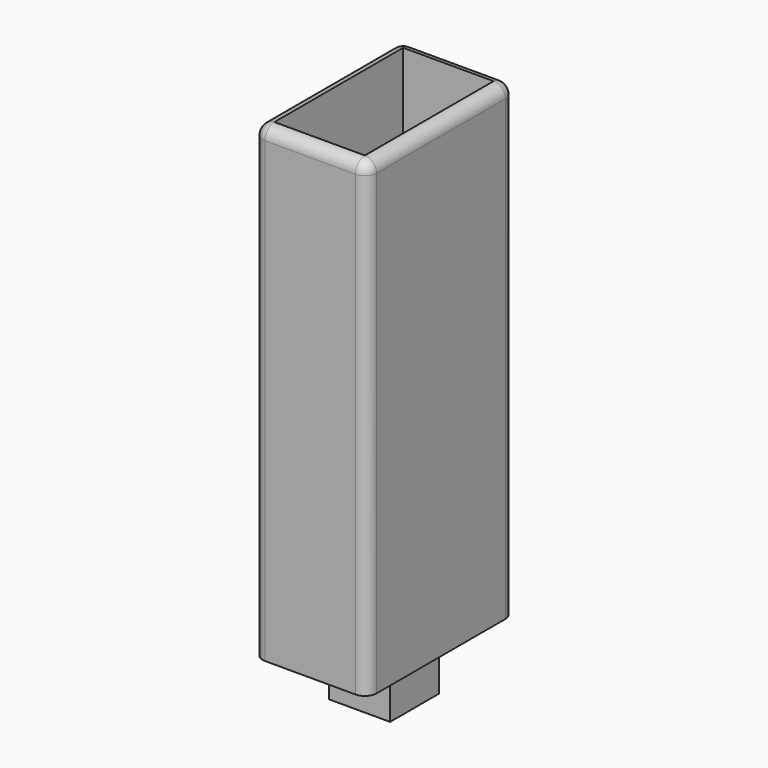
from build123d import *

# Parameters (mm, degrees)
F0_W     = 12.319
F0_H     = 19.939
F1_DEPTH = 50.8
F2_T     = -1.27
F3_R     = 1.26999
F4_W     = 6.604
F4_H     = 6.604
F5_DEPTH = 5.842


# Not quite as in the source:
# - a fillet or chamfer is up to 0.001 mm smaller than in the source, because OpenCascade refuses the exact size


with BuildPart() as f1:
    # F0 (on Top) → F1 (new body)
    with BuildSketch(Plane.XY):
        Rectangle(F0_W, F0_H)
    extrude(amount=F1_DEPTH)

    # F2
    f2_openings = [f1.faces().sort_by_distance(p)[0] for p in [
        (0, 0, 50.8),
    ]]
    offset(amount=F2_T, openings=f2_openings)

    # F3 (radius 1.27 in the source; OpenCascade refuses exactly that, so slightly less here)
    f3_edges = [f1.edges().sort_by_distance(p)[0] for p in [
        (0, -9.9695, 50.8),
        (6.1595, 0, 50.8),
        (0, 9.9695, 50.8),
        (-6.1595, 0, 50.8),
        (-6.1595, -9.9695, 25.4),
        (6.1595, -9.9695, 25.4),
        (6.1595, 9.9695, 25.4),
        (-6.1595, 9.9695, 25.4),
    ]]
    fillet(f3_edges, radius=F3_R)

    # F4 (on face) → F5 (join)
    with BuildSketch(Plane(origin=(0, 0, 0), x_dir=(1, 0, 0), z_dir=(0, 0, -1))):
        Rectangle(F4_W, F4_H)
    extrude(amount=F5_DEPTH)


solid = f1.part
